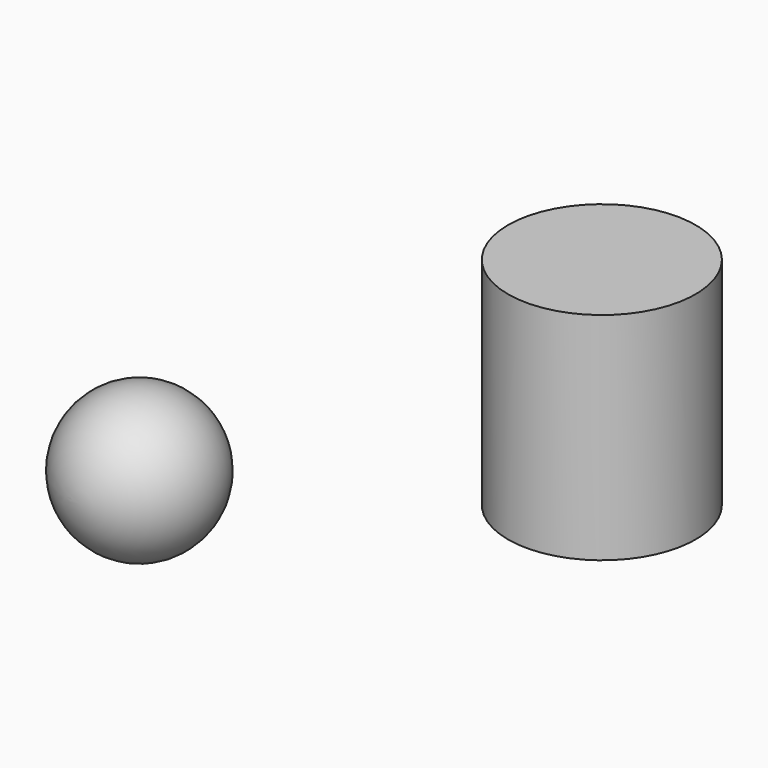
from build123d import *

# Parameters (mm, degrees)
F0_W = 14.327137731
F0_H = 32.9927764833


# Not quite as in the source:
# - the program builds the solid bodies; features that only make, move or delete a surface that nothing else refers to are left out


with BuildPart() as f1:
    # F0 (on Front) → F1 (revolve)
    with BuildSketch(Plane.XZ):
        with Locations((-7.1635688655, 16.4963882416)):
            Rectangle(F0_W, F0_H)
    revolve(axis=Axis((0, 0, 16.4963882416), (0, 0, -1)))


with BuildPart() as f3:
    # F2 (on Top) → F3 (revolve)
    with BuildSketch(Plane.XY):
        with BuildLine():
            Line((-48.6315526068, -27.5444276631), (-48.6315526068, -16.4001730611))
            ThreePointArc((-48.6315526068, -16.4001730611), (-59.7758072088, -27.5444276631), (-48.6315526068, -38.688682265))
            Line((-48.6315526068, -38.688682265), (-48.6315526068, -27.5444276631))
        make_face()
    revolve(axis=Axis((-48.6315526068, -27.5444276631, 0), (0, 1, 0)))


solid = Compound([f1.part, f3.part])
